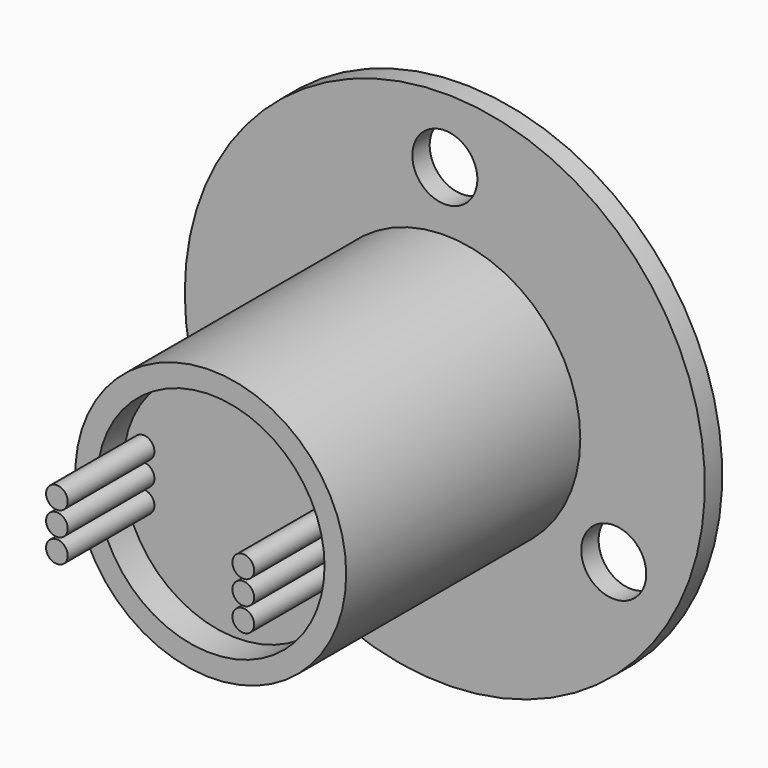
from build123d import *

# Parameters (mm, degrees)
F0_R      = 6.25
F1_DEPTH  = 13.5
F2_R      = 12
F2_R_2    = 1.5
F2_R_3    = 6.25
F3_DEPTH  = 1
F4_R      = 5.5
F4_R_2    = 2.5
F5_DEPTH  = 1
F6_DEPTH  = 3
F7_R      = 3
F7_R_2    = 2.5
F8_DEPTH  = 1
F9_R      = 5.25
F10_DEPTH = 1.5
F11_R     = 0.5
F12_DEPTH = 5
F13_R     = 0.5
F14_DEPTH = 5


with BuildPart() as f1:
    # F0 (on Front) → F1 (new body)
    with BuildSketch(Plane.XZ):
        Circle(F0_R)
    extrude(amount=F1_DEPTH)

    # F2 (on face) → F3 (join)
    with BuildSketch(Plane(origin=(0, 0, 0), x_dir=(-1, 0, 0), z_dir=(0, 1, 0))):
        Circle(F2_R)
        with Locations((-7.7942286341, -4.5)):
            Circle(F2_R_2, mode=Mode.SUBTRACT)
        with Locations((7.7942286341, -4.5)):
            Circle(F2_R_2, mode=Mode.SUBTRACT)
        Circle(F2_R_3, mode=Mode.SUBTRACT)
        with Locations((0, 9)):
            Circle(F2_R_2, mode=Mode.SUBTRACT)
        Circle(F2_R_3)
    extrude(amount=F3_DEPTH)

    # F4 (on face) → F5 (join)
    with BuildSketch(Plane(origin=(0, 1, 0), x_dir=(-1, 0, 0), z_dir=(0, 1, 0))):
        Circle(F4_R)
        Circle(F4_R_2, mode=Mode.SUBTRACT)
    extrude(amount=F5_DEPTH)

    # F6 (add): a face of the model
    f6_faces = [f1.faces().sort_by_distance(p)[0] for p in [
        (0, 1, 0),
    ]]
    extrude(f6_faces, amount=F6_DEPTH)

    # F7 (on face) → F8 (cut)
    with BuildSketch(Plane(origin=(0, 2, 0), x_dir=(-1, 0, 0), z_dir=(0, 1, 0))):
        Circle(F7_R)
        Circle(F7_R_2, mode=Mode.SUBTRACT)
    extrude(amount=-F8_DEPTH, mode=Mode.SUBTRACT)

    # F9 (on face) → F10 (cut)
    with BuildSketch(Plane.XZ.offset(13.5)):
        Circle(F9_R)
    extrude(amount=-F10_DEPTH, mode=Mode.SUBTRACT)

    # F11 (on face) → F12 (join)
    with BuildSketch(Plane.XZ.offset(12)):
        with Locations((-4.3, -1.1)):
            Circle(F11_R)
        with Locations((-4.3, 0)):
            Circle(F11_R)
        with Locations((-4.3, 1.1)):
            Circle(F11_R)
        with Locations((4.3, 1.1)):
            Circle(F11_R)
        with Locations((4.3, 0)):
            Circle(F11_R)
        with Locations((4.3, -1.1)):
            Circle(F11_R)
    extrude(amount=F12_DEPTH)

    # F13 (on face) → F14 (join)
    with BuildSketch(Plane(origin=(0, 4, 0), x_dir=(-1, 0, 0), z_dir=(0, 1, 0))):
        with Locations((-0.875, -1.5155444566)):
            Circle(F13_R)
        with Locations((0.875, -1.5155444566)):
            Circle(F13_R)
        with Locations((1.75, 0)):
            Circle(F13_R)
        with Locations((0.875, 1.5155444566)):
            Circle(F13_R)
        with Locations((-0.875, 1.5155444566)):
            Circle(F13_R)
        with Locations((-1.75, 0)):
            Circle(F13_R)
    extrude(amount=F14_DEPTH)


solid = f1.part
